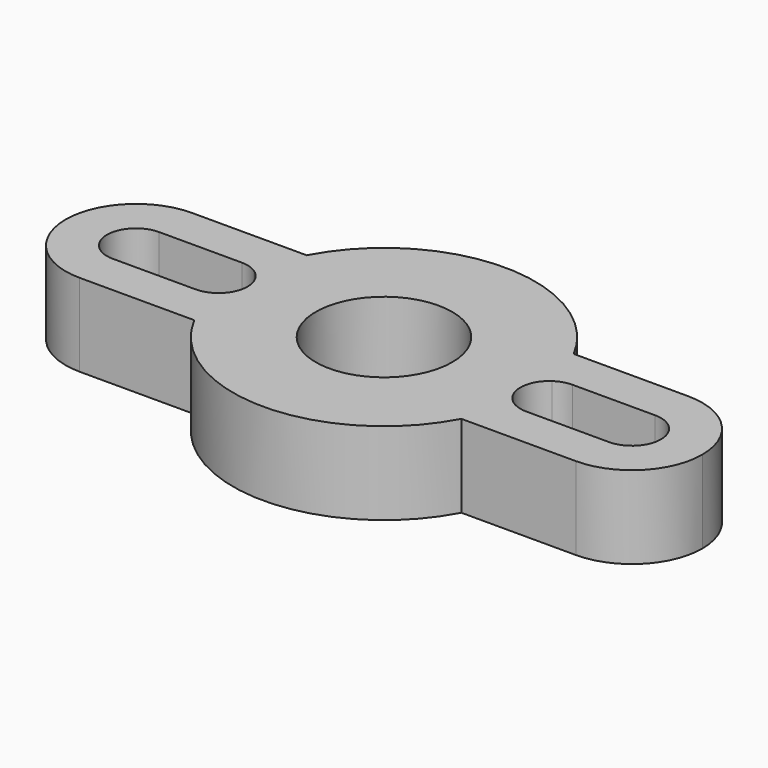
from build123d import *

# Parameters (mm, degrees)
F0_R     = 4.125
F1_DEPTH = 5
F2_DEPTH = 5
F3_DEPTH = 5
F4_DEPTH = 5
F5_DEPTH = 25
F6_DEPTH = 25


with BuildPart() as f1:
    # F0 (on Top) → F1 (new body)
    with BuildSketch(Plane.XY):
        with BuildLine():
            Line((-8.0748451998, 4.25), (8.0748451998, 4.25))
            ThreePointArc((8.0748451998, 4.25), (0, 9.125), (-8.0748451998, 4.25))
        make_face()
        with BuildLine():
            ThreePointArc((8.26015625, -3.8775564117), (5.75, 0), (8.26015625, 3.8775564117))
            ThreePointArc((8.26015625, 3.8775564117), (8.1696234092, 4.0648343573), (8.0748451998, 4.25))
            Line((8.0748451998, 4.25), (-8.0748451998, 4.25))
            ThreePointArc((-8.0748451998, 4.25), (-8.1696234092, 4.0648343573), (-8.26015625, 3.8775564117))
            ThreePointArc((-8.26015625, 3.8775564117), (-6.4323091545, 2.3095631689), (-5.75, 0))
            ThreePointArc((-5.75, 0), (-6.4323091545, -2.3095631689), (-8.26015625, -3.8775564117))
            ThreePointArc((-8.26015625, -3.8775564117), (-8.1696234092, -4.0648343573), (-8.0748451998, -4.25))
            Line((-8.0748451998, -4.25), (8.0748451998, -4.25))
            ThreePointArc((8.0748451998, -4.25), (8.1696234092, -4.0648343573), (8.26015625, -3.8775564117))
        make_face()
        Circle(F0_R, mode=Mode.SUBTRACT)
        with BuildLine():
            ThreePointArc((-8.0748451998, -4.25), (0, -9.125), (8.0748451998, -4.25))
            Line((8.0748451998, -4.25), (-8.0748451998, -4.25))
        make_face()
        with BuildLine():
            ThreePointArc((-5.75, 0), (-6.4323091545, 2.3095631689), (-8.26015625, 3.8775564117))
            ThreePointArc((-8.26015625, 3.8775564117), (-8.7205215176, 2.6866576746), (-9.01015625, 1.4431595028))
            ThreePointArc((-9.01015625, 1.4431595028), (-8.4516578927, 0.8155591449), (-8.25, 0))
            ThreePointArc((-8.25, 0), (-8.4516578927, -0.8155591449), (-9.01015625, -1.4431595028))
            ThreePointArc((-9.01015625, -1.4431595028), (-8.7205215176, -2.6866576746), (-8.26015625, -3.8775564117))
            ThreePointArc((-8.26015625, -3.8775564117), (-6.4323091545, -2.3095631689), (-5.75, 0))
        make_face()
        with BuildLine():
            ThreePointArc((-9.01015625, 1.4431595028), (-8.7205215176, 2.6866576746), (-8.26015625, 3.8775564117))
            ThreePointArc((-8.26015625, 3.8775564117), (-9.1103693883, 4.1558461683), (-10, 4.25))
            ThreePointArc((-10, 4.25), (-11.3144466464, 4.041624675), (-12.5, 3.4369317712))
            ThreePointArc((-12.5, 3.4369317712), (-11.703765196, 2.6827851418), (-11.1270166538, 1.75))
            Line((-11.1270166538, 1.75), (-10, 1.75))
            ThreePointArc((-10, 1.75), (-9.4818441981, 1.6715306055), (-9.01015625, 1.4431595028))
        make_face()
        with BuildLine():
            ThreePointArc((-12.5, 3.4369317712), (-11.3144466464, 4.041624675), (-10, 4.25))
            Line((-10, 4.25), (-15, 4.25))
            ThreePointArc((-15, 4.25), (-13.6855533536, 4.041624675), (-12.5, 3.4369317712))
        make_face()
        with BuildLine():
            ThreePointArc((-13.8729833462, 1.75), (-13.296234804, 2.6827851418), (-12.5, 3.4369317712))
            ThreePointArc((-12.5, 3.4369317712), (-13.6855533536, 4.041624675), (-15, 4.25))
            Line((-15, 4.25), (-15, 1.75))
            Line((-15, 1.75), (-13.8729833462, 1.75))
        make_face()
        with BuildLine():
            Line((-15, 1.75), (-15, 4.25))
            ThreePointArc((-15, 4.25), (-19.25, 0), (-15, -4.25))
            Line((-15, -4.25), (-15, -1.75))
            ThreePointArc((-15, -1.75), (-16.75, 0), (-15, 1.75))
        make_face()
        with BuildLine():
            ThreePointArc((-11.1270166538, 1.75), (-11.703765196, 2.6827851418), (-12.5, 3.4369317712))
            ThreePointArc((-12.5, 3.4369317712), (-13.296234804, 2.6827851418), (-13.8729833462, 1.75))
            Line((-13.8729833462, 1.75), (-11.1270166538, 1.75))
        make_face()
        with BuildLine():
            ThreePointArc((-11, 1.4361406616), (-11.0603815396, 1.5943357195), (-11.1270166538, 1.75))
            Line((-11.1270166538, 1.75), (-13.8729833462, 1.75))
            ThreePointArc((-13.8729833462, 1.75), (-13.9396184604, 1.5943357195), (-14, 1.4361406616))
            ThreePointArc((-14, 1.4361406616), (-13.4487907943, 0.8100925873), (-13.25, 0))
            ThreePointArc((-13.25, 0), (-13.4487907943, -0.8100925873), (-14, -1.4361406616))
            ThreePointArc((-14, -1.4361406616), (-13.9396184604, -1.5943357195), (-13.8729833462, -1.75))
            Line((-13.8729833462, -1.75), (-11.1270166538, -1.75))
            ThreePointArc((-11.1270166538, -1.75), (-11.0603815396, -1.5943357195), (-11, -1.4361406616))
            ThreePointArc((-11, -1.4361406616), (-11.75, 0), (-11, 1.4361406616))
        make_face()
        with BuildLine():
            ThreePointArc((-15, -4.25), (-13.6855533536, -4.041624675), (-12.5, -3.4369317712))
            ThreePointArc((-12.5, -3.4369317712), (-13.296234804, -2.6827851418), (-13.8729833462, -1.75))
            Line((-13.8729833462, -1.75), (-15, -1.75))
            Line((-15, -1.75), (-15, -4.25))
        make_face()
        with BuildLine():
            ThreePointArc((-13.8729833462, -1.75), (-13.296234804, -2.6827851418), (-12.5, -3.4369317712))
            ThreePointArc((-12.5, -3.4369317712), (-11.703765196, -2.6827851418), (-11.1270166538, -1.75))
            Line((-11.1270166538, -1.75), (-13.8729833462, -1.75))
        make_face()
        with BuildLine():
            ThreePointArc((-10, -4.25), (-9.1103693883, -4.1558461683), (-8.26015625, -3.8775564117))
            ThreePointArc((-8.26015625, -3.8775564117), (-8.7205215176, -2.6866576746), (-9.01015625, -1.4431595028))
            ThreePointArc((-9.01015625, -1.4431595028), (-9.4818441981, -1.6715306055), (-10, -1.75))
            Line((-10, -1.75), (-11.1270166538, -1.75))
            ThreePointArc((-11.1270166538, -1.75), (-11.703765196, -2.6827851418), (-12.5, -3.4369317712))
            ThreePointArc((-12.5, -3.4369317712), (-11.3144466464, -4.041624675), (-10, -4.25))
        make_face()
        with BuildLine():
            Line((-15, -4.25), (-10, -4.25))
            ThreePointArc((-10, -4.25), (-11.3144466464, -4.041624675), (-12.5, -3.4369317712))
            ThreePointArc((-12.5, -3.4369317712), (-13.6855533536, -4.041624675), (-15, -4.25))
        make_face()
        with BuildLine():
            ThreePointArc((-14, 1.4361406616), (-13.9396184604, 1.5943357195), (-13.8729833462, 1.75))
            Line((-13.8729833462, 1.75), (-15, 1.75))
            ThreePointArc((-15, 1.75), (-14.4759514134, 1.6696925103), (-14, 1.4361406616))
        make_face()
        with BuildLine():
            ThreePointArc((-11, 1.4361406616), (-10.5240485866, 1.6696925103), (-10, 1.75))
            Line((-10, 1.75), (-11.1270166538, 1.75))
            ThreePointArc((-11.1270166538, 1.75), (-11.0603815396, 1.5943357195), (-11, 1.4361406616))
        make_face()
        with BuildLine():
            Line((-15, -1.75), (-13.8729833462, -1.75))
            ThreePointArc((-13.8729833462, -1.75), (-13.9396184604, -1.5943357195), (-14, -1.4361406616))
            ThreePointArc((-14, -1.4361406616), (-14.4759514134, -1.6696925103), (-15, -1.75))
        make_face()
        with BuildLine():
            Line((-11.1270166538, -1.75), (-10, -1.75))
            ThreePointArc((-10, -1.75), (-10.5240485866, -1.6696925103), (-11, -1.4361406616))
            ThreePointArc((-11, -1.4361406616), (-11.0603815396, -1.5943357195), (-11.1270166538, -1.75))
        make_face()
    extrude(amount=F1_DEPTH)



with BuildPart() as f1b:
    # F0 (on Top) → F1, piece 2 (new body)
    with BuildSketch(Plane.XY):
        with BuildLine():
            Line((15, 4.25), (15, 1.75))
            ThreePointArc((15, 1.75), (16.2374368671, 1.2374368671), (16.75, 0))
            ThreePointArc((16.75, 0), (16.2374368671, -1.2374368671), (15, -1.75))
            Line((15, -1.75), (15, -4.25))
            ThreePointArc((15, -4.25), (18.00520382, -3.00520382), (19.25, 0))
            ThreePointArc((19.25, 0), (18.00520382, 3.00520382), (15, 4.25))
        make_face()
    extrude(amount=F1_DEPTH)


with BuildPart() as f1c:
    # F0 (on Top) → F1, piece 3 (new body)
    with BuildSketch(Plane.XY):
        with BuildLine():
            ThreePointArc((12.5, 3.4369317712), (11.703765196, 2.6827851418), (11.1270166538, 1.75))
            Line((11.1270166538, 1.75), (13.8729833462, 1.75))
            ThreePointArc((13.8729833462, 1.75), (13.296234804, 2.6827851418), (12.5, 3.4369317712))
        make_face()
        with BuildLine():
            ThreePointArc((11, 1.4361406616), (11.5512092057, 0.8100925873), (11.75, 0))
            ThreePointArc((11.75, 0), (11.5512092057, -0.8100925873), (11, -1.4361406616))
            ThreePointArc((11, -1.4361406616), (11.0603815396, -1.5943357195), (11.1270166538, -1.75))
            Line((11.1270166538, -1.75), (13.8729833462, -1.75))
            ThreePointArc((13.8729833462, -1.75), (13.9396184604, -1.5943357195), (14, -1.4361406616))
            ThreePointArc((14, -1.4361406616), (13.25, 0), (14, 1.4361406616))
            ThreePointArc((14, 1.4361406616), (13.9396184604, 1.5943357195), (13.8729833462, 1.75))
            Line((13.8729833462, 1.75), (11.1270166538, 1.75))
            ThreePointArc((11.1270166538, 1.75), (11.0603815396, 1.5943357195), (11, 1.4361406616))
        make_face()
        with BuildLine():
            ThreePointArc((14, -1.4361406616), (13.9396184604, -1.5943357195), (13.8729833462, -1.75))
            Line((13.8729833462, -1.75), (15, -1.75))
            ThreePointArc((15, -1.75), (14.4759514134, -1.6696925103), (14, -1.4361406616))
        make_face()
        with BuildLine():
            Line((15, 1.75), (13.8729833462, 1.75))
            ThreePointArc((13.8729833462, 1.75), (13.9396184604, 1.5943357195), (14, 1.4361406616))
            ThreePointArc((14, 1.4361406616), (14.4759514134, 1.6696925103), (15, 1.75))
        make_face()
    extrude(amount=F1_DEPTH)


with BuildPart() as f1_1:
    add(f1.part)

    add(f1b.part)  # F2 merges F1b

    add(f1c.part)  # F2 merges F1c
    # F0 (on Top) → F2 (join)
    with BuildSketch(Plane.XY):
        with BuildLine():
            ThreePointArc((12.5, 3.4369317712), (13.296234804, 2.6827851418), (13.8729833462, 1.75))
            Line((13.8729833462, 1.75), (15, 1.75))
            Line((15, 1.75), (15, 4.25))
            ThreePointArc((15, 4.25), (13.6855533536, 4.041624675), (12.5, 3.4369317712))
        make_face()
        with BuildLine():
            ThreePointArc((10, 4.25), (11.3144466464, 4.041624675), (12.5, 3.4369317712))
            ThreePointArc((12.5, 3.4369317712), (13.6855533536, 4.041624675), (15, 4.25))
            Line((15, 4.25), (10, 4.25))
        make_face()
        with BuildLine():
            ThreePointArc((9.01015625, 1.4431595028), (9.4818441981, 1.6715306055), (10, 1.75))
            Line((10, 1.75), (11.1270166538, 1.75))
            ThreePointArc((11.1270166538, 1.75), (11.703765196, 2.6827851418), (12.5, 3.4369317712))
            ThreePointArc((12.5, 3.4369317712), (11.3144466464, 4.041624675), (10, 4.25))
            ThreePointArc((10, 4.25), (9.1103693883, 4.1558461683), (8.26015625, 3.8775564117))
            ThreePointArc((8.26015625, 3.8775564117), (8.7205215176, 2.6866576746), (9.01015625, 1.4431595028))
        make_face()
        with BuildLine():
            ThreePointArc((9.01015625, -1.4431595028), (8.25, 0), (9.01015625, 1.4431595028))
            ThreePointArc((9.01015625, 1.4431595028), (8.7205215176, 2.6866576746), (8.26015625, 3.8775564117))
            ThreePointArc((8.26015625, 3.8775564117), (5.75, 0), (8.26015625, -3.8775564117))
            ThreePointArc((8.26015625, -3.8775564117), (8.7205215176, -2.6866576746), (9.01015625, -1.4431595028))
        make_face()
        with BuildLine():
            Line((15, -1.75), (13.8729833462, -1.75))
            ThreePointArc((13.8729833462, -1.75), (13.296234804, -2.6827851418), (12.5, -3.4369317712))
            ThreePointArc((12.5, -3.4369317712), (13.6855533536, -4.041624675), (15, -4.25))
            Line((15, -4.25), (15, -1.75))
        make_face()
        with BuildLine():
            ThreePointArc((15, -4.25), (13.6855533536, -4.041624675), (12.5, -3.4369317712))
            ThreePointArc((12.5, -3.4369317712), (11.3144466464, -4.041624675), (10, -4.25))
            Line((10, -4.25), (15, -4.25))
        make_face()
        with BuildLine():
            Line((11.1270166538, -1.75), (10, -1.75))
            ThreePointArc((10, -1.75), (9.4818441981, -1.6715306055), (9.01015625, -1.4431595028))
            ThreePointArc((9.01015625, -1.4431595028), (8.7205215176, -2.6866576746), (8.26015625, -3.8775564117))
            ThreePointArc((8.26015625, -3.8775564117), (9.1103693883, -4.1558461683), (10, -4.25))
            ThreePointArc((10, -4.25), (11.3144466464, -4.041624675), (12.5, -3.4369317712))
            ThreePointArc((12.5, -3.4369317712), (11.703765196, -2.6827851418), (11.1270166538, -1.75))
        make_face()
        with BuildLine():
            Line((13.8729833462, -1.75), (11.1270166538, -1.75))
            ThreePointArc((11.1270166538, -1.75), (11.703765196, -2.6827851418), (12.5, -3.4369317712))
            ThreePointArc((12.5, -3.4369317712), (13.296234804, -2.6827851418), (13.8729833462, -1.75))
        make_face()
        with BuildLine():
            ThreePointArc((10, 1.75), (10.5240485866, 1.6696925103), (11, 1.4361406616))
            ThreePointArc((11, 1.4361406616), (11.0603815396, 1.5943357195), (11.1270166538, 1.75))
            Line((11.1270166538, 1.75), (10, 1.75))
        make_face()
        with BuildLine():
            ThreePointArc((11.1270166538, -1.75), (11.0603815396, -1.5943357195), (11, -1.4361406616))
            ThreePointArc((11, -1.4361406616), (10.5240485866, -1.6696925103), (10, -1.75))
            Line((10, -1.75), (11.1270166538, -1.75))
        make_face()
    extrude(amount=F2_DEPTH)

    # F0 (on Top) → F3 (join)
    with BuildSketch(Plane.XY):
        with BuildLine():
            ThreePointArc((8.0748451998, 4.25), (8.1696234092, 4.0648343573), (8.26015625, 3.8775564117))
            ThreePointArc((8.26015625, 3.8775564117), (9.1103693883, 4.1558461683), (10, 4.25))
            Line((10, 4.25), (8.0748451998, 4.25))
        make_face()
        with BuildLine():
            ThreePointArc((10, -4.25), (9.1103693883, -4.1558461683), (8.26015625, -3.8775564117))
            ThreePointArc((8.26015625, -3.8775564117), (8.1696234092, -4.0648343573), (8.0748451998, -4.25))
            Line((8.0748451998, -4.25), (10, -4.25))
        make_face()
        with BuildLine():
            Line((-10, -4.25), (-8.0748451998, -4.25))
            ThreePointArc((-8.0748451998, -4.25), (-8.1696234092, -4.0648343573), (-8.26015625, -3.8775564117))
            ThreePointArc((-8.26015625, -3.8775564117), (-9.1103693883, -4.1558461683), (-10, -4.25))
        make_face()
        with BuildLine():
            ThreePointArc((-8.26015625, 3.8775564117), (-8.1696234092, 4.0648343573), (-8.0748451998, 4.25))
            Line((-8.0748451998, 4.25), (-10, 4.25))
            ThreePointArc((-10, 4.25), (-9.1103693883, 4.1558461683), (-8.26015625, 3.8775564117))
        make_face()
    extrude(amount=F3_DEPTH)

    # F0 (on Top) → F4 (join)
    with BuildSketch(Plane.XY):
        with BuildLine():
            ThreePointArc((11, -1.4361406616), (11.5512092057, -0.8100925873), (11.75, 0))
            ThreePointArc((11.75, 0), (11.5512092057, 0.8100925873), (11, 1.4361406616))
            ThreePointArc((11, 1.4361406616), (10.75, 0), (11, -1.4361406616))
        make_face()
        with BuildLine():
            Line((10, -1.75), (10, 1.75))
            ThreePointArc((10, 1.75), (9.4818441981, 1.6715306055), (9.01015625, 1.4431595028))
            ThreePointArc((9.01015625, 1.4431595028), (9.0962437517, 0.7238609047), (9.125, 0))
            ThreePointArc((9.125, 0), (9.0962437517, -0.7238609047), (9.01015625, -1.4431595028))
            ThreePointArc((9.01015625, -1.4431595028), (9.4818441981, -1.6715306055), (10, -1.75))
        make_face()
        with BuildLine():
            ThreePointArc((9.125, 0), (9.0962437517, 0.7238609047), (9.01015625, 1.4431595028))
            ThreePointArc((9.01015625, 1.4431595028), (8.25, 0), (9.01015625, -1.4431595028))
            ThreePointArc((9.01015625, -1.4431595028), (9.0962437517, -0.7238609047), (9.125, 0))
        make_face()
        with BuildLine():
            ThreePointArc((11, -1.4361406616), (10.75, 0), (11, 1.4361406616))
            ThreePointArc((11, 1.4361406616), (10.5240485866, 1.6696925103), (10, 1.75))
            Line((10, 1.75), (10, -1.75))
            ThreePointArc((10, -1.75), (10.5240485866, -1.6696925103), (11, -1.4361406616))
        make_face()
    extrude(amount=F4_DEPTH)

    # F0 (on Top) → F5 (cut)
    with BuildSketch(Plane.XY):
        with BuildLine():
            ThreePointArc((-11, 1.4361406616), (-11.0603815396, 1.5943357195), (-11.1270166538, 1.75))
            Line((-11.1270166538, 1.75), (-13.8729833462, 1.75))
            ThreePointArc((-13.8729833462, 1.75), (-13.9396184604, 1.5943357195), (-14, 1.4361406616))
            ThreePointArc((-14, 1.4361406616), (-13.4487907943, 0.8100925873), (-13.25, 0))
            ThreePointArc((-13.25, 0), (-13.4487907943, -0.8100925873), (-14, -1.4361406616))
            ThreePointArc((-14, -1.4361406616), (-13.9396184604, -1.5943357195), (-13.8729833462, -1.75))
            Line((-13.8729833462, -1.75), (-11.1270166538, -1.75))
            ThreePointArc((-11.1270166538, -1.75), (-11.0603815396, -1.5943357195), (-11, -1.4361406616))
            ThreePointArc((-11, -1.4361406616), (-11.75, 0), (-11, 1.4361406616))
        make_face()
        with BuildLine():
            Line((-15, -1.75), (-13.8729833462, -1.75))
            ThreePointArc((-13.8729833462, -1.75), (-13.9396184604, -1.5943357195), (-14, -1.4361406616))
            ThreePointArc((-14, -1.4361406616), (-14.4759514134, -1.6696925103), (-15, -1.75))
        make_face()
        with BuildLine():
            ThreePointArc((-14, 1.4361406616), (-13.9396184604, 1.5943357195), (-13.8729833462, 1.75))
            Line((-13.8729833462, 1.75), (-15, 1.75))
            ThreePointArc((-15, 1.75), (-14.4759514134, 1.6696925103), (-14, 1.4361406616))
        make_face()
        with BuildLine():
            ThreePointArc((-11, 1.4361406616), (-10.5240485866, 1.6696925103), (-10, 1.75))
            Line((-10, 1.75), (-11.1270166538, 1.75))
            ThreePointArc((-11.1270166538, 1.75), (-11.0603815396, 1.5943357195), (-11, 1.4361406616))
        make_face()
        with BuildLine():
            Line((-11.1270166538, -1.75), (-10, -1.75))
            ThreePointArc((-10, -1.75), (-10.5240485866, -1.6696925103), (-11, -1.4361406616))
            ThreePointArc((-11, -1.4361406616), (-11.0603815396, -1.5943357195), (-11.1270166538, -1.75))
        make_face()
    extrude(amount=F5_DEPTH, mode=Mode.SUBTRACT)

    # F0 (on Top) → F6 (cut)
    with BuildSketch(Plane.XY):
        with BuildLine():
            ThreePointArc((9.125, 0), (9.0962437517, 0.7238609047), (9.01015625, 1.4431595028))
            ThreePointArc((9.01015625, 1.4431595028), (8.25, 0), (9.01015625, -1.4431595028))
            ThreePointArc((9.01015625, -1.4431595028), (9.0962437517, -0.7238609047), (9.125, 0))
        make_face()
        with BuildLine():
            Line((10, -1.75), (10, 1.75))
            ThreePointArc((10, 1.75), (9.4818441981, 1.6715306055), (9.01015625, 1.4431595028))
            ThreePointArc((9.01015625, 1.4431595028), (9.0962437517, 0.7238609047), (9.125, 0))
            ThreePointArc((9.125, 0), (9.0962437517, -0.7238609047), (9.01015625, -1.4431595028))
            ThreePointArc((9.01015625, -1.4431595028), (9.4818441981, -1.6715306055), (10, -1.75))
        make_face()
        with BuildLine():
            ThreePointArc((11, -1.4361406616), (10.75, 0), (11, 1.4361406616))
            ThreePointArc((11, 1.4361406616), (10.5240485866, 1.6696925103), (10, 1.75))
            Line((10, 1.75), (10, -1.75))
            ThreePointArc((10, -1.75), (10.5240485866, -1.6696925103), (11, -1.4361406616))
        make_face()
        with BuildLine():
            ThreePointArc((11, -1.4361406616), (11.5512092057, -0.8100925873), (11.75, 0))
            ThreePointArc((11.75, 0), (11.5512092057, 0.8100925873), (11, 1.4361406616))
            ThreePointArc((11, 1.4361406616), (10.75, 0), (11, -1.4361406616))
        make_face()
        with BuildLine():
            ThreePointArc((11.1270166538, -1.75), (11.0603815396, -1.5943357195), (11, -1.4361406616))
            ThreePointArc((11, -1.4361406616), (10.5240485866, -1.6696925103), (10, -1.75))
            Line((10, -1.75), (11.1270166538, -1.75))
        make_face()
        with BuildLine():
            ThreePointArc((10, 1.75), (10.5240485866, 1.6696925103), (11, 1.4361406616))
            ThreePointArc((11, 1.4361406616), (11.0603815396, 1.5943357195), (11.1270166538, 1.75))
            Line((11.1270166538, 1.75), (10, 1.75))
        make_face()
        with BuildLine():
            ThreePointArc((14, -1.4361406616), (13.9396184604, -1.5943357195), (13.8729833462, -1.75))
            Line((13.8729833462, -1.75), (15, -1.75))
            ThreePointArc((15, -1.75), (14.4759514134, -1.6696925103), (14, -1.4361406616))
        make_face()
        with BuildLine():
            Line((15, 1.75), (13.8729833462, 1.75))
            ThreePointArc((13.8729833462, 1.75), (13.9396184604, 1.5943357195), (14, 1.4361406616))
            ThreePointArc((14, 1.4361406616), (14.4759514134, 1.6696925103), (15, 1.75))
        make_face()
        with BuildLine():
            ThreePointArc((11, 1.4361406616), (11.5512092057, 0.8100925873), (11.75, 0))
            ThreePointArc((11.75, 0), (11.5512092057, -0.8100925873), (11, -1.4361406616))
            ThreePointArc((11, -1.4361406616), (11.0603815396, -1.5943357195), (11.1270166538, -1.75))
            Line((11.1270166538, -1.75), (13.8729833462, -1.75))
            ThreePointArc((13.8729833462, -1.75), (13.9396184604, -1.5943357195), (14, -1.4361406616))
            ThreePointArc((14, -1.4361406616), (13.25, 0), (14, 1.4361406616))
            ThreePointArc((14, 1.4361406616), (13.9396184604, 1.5943357195), (13.8729833462, 1.75))
            Line((13.8729833462, 1.75), (11.1270166538, 1.75))
            ThreePointArc((11.1270166538, 1.75), (11.0603815396, 1.5943357195), (11, 1.4361406616))
        make_face()
    extrude(amount=F6_DEPTH, mode=Mode.SUBTRACT)


solid = f1_1.part
